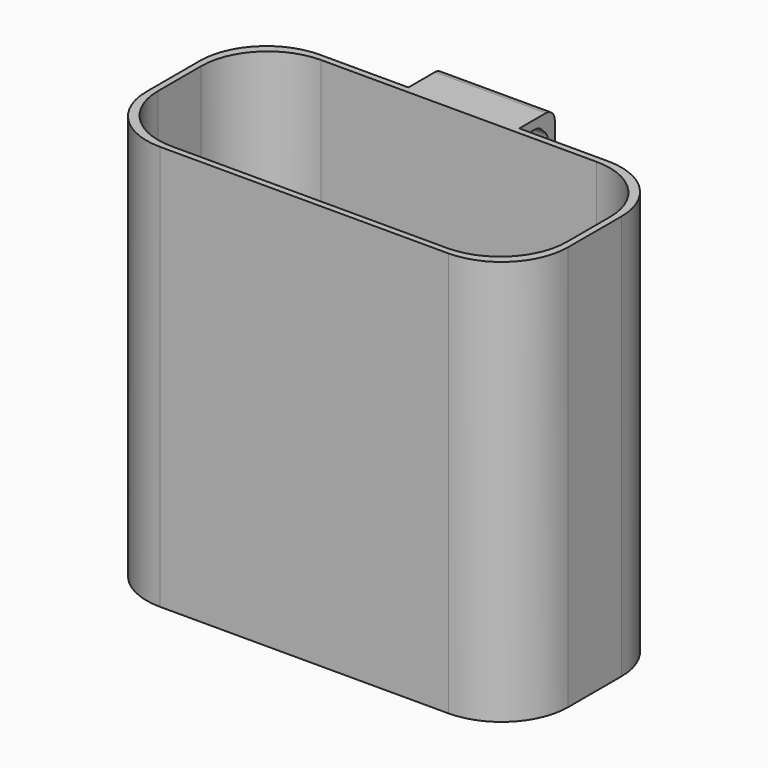
from build123d import *

# Parameters (mm, degrees)
F0_W          = 95
F0_H          = 45
F1_DEPTH      = 1.28
F2_W          = 95
F2_H          = 45
F2_W_2        = 92.12
F2_H_2        = 42.12
F3_DEPTH      = 90
F4_W          = 25
F4_H          = 35
F5_DEPTH      = 10
F6_W          = 8
F6_H          = 31
F7_DEPTH      = 60.001
F9_DEPTH      = 25
F11_DEPTH     = 10
F12_SIZE      = 2.5
F13_T1_DEPTH  = 25
F13_T3_DEPTH  = 37.5
F13_T5_DEPTH  = 28.3493649054
F13_T10_DEPTH = 35.1683904211
F13_T15_DEPTH = 35.1683904211
F14_R         = 15
F15_R         = 15
F16_R         = 15


# Not quite as in the source:
# - a fillet or chamfer that OpenCascade refuses, or shapes differently, is made with other operations: its cross-section is extruded or revolved along the edge and cut away or added


with BuildPart() as f1:
    # F0 (on Top) → F1 (new body)
    with BuildSketch(Plane.XY):
        with Locations((47.5, 22.5)):
            Rectangle(F0_W, F0_H)
    extrude(amount=F1_DEPTH)

    # F2 (on face) → F3 (join)
    with BuildSketch(Plane.XY.offset(1.28)):
        with Locations((47.5, 22.5)):
            Rectangle(F2_W, F2_H)
        with Locations((47.5, 22.5)):
            Rectangle(F2_W_2, F2_H_2, mode=Mode.SUBTRACT)
    extrude(amount=F3_DEPTH)

    # F4 (on face) → F5 (join)
    with BuildSketch(Plane(origin=(0, 45, 0), x_dir=(-1, 0, 0), z_dir=(0, 1, 0))):
        with Locations((-47.5, 73.78)):
            Rectangle(F4_W, F4_H)
    extrude(amount=F5_DEPTH)

    # F6 (on face) → F7 (cut, through all)
    with BuildSketch(Plane.YZ.offset(60)):
        with Locations((49, 73.78)):
            Rectangle(F6_W, F6_H)
    extrude(amount=-F7_DEPTH, mode=Mode.SUBTRACT)

    # F8 (on face) → F9 (join, through all)
    with BuildSketch(Plane.YZ.offset(60)):
        Polygon((55, 56.28), (45, 56.28), (45, 38.9594919243), align=None)
    extrude(amount=-F9_DEPTH)

    # F10 (on face) → F11 (cut, through all)
    with BuildSketch(Plane(origin=(0, 55, 0), x_dir=(-1, 0, 0), z_dir=(0, 1, 0))):
        Polygon((-53.6958506181, 38.9594919243), (-60, 56.28), (-60, 38.9594919243), align=None)
        Polygon((-41.304149382, 38.9594919243), (-35, 38.9594919243), (-35, 56.28), align=None)
    extrude(amount=-F11_DEPTH, mode=Mode.SUBTRACT)

    # F12
    f12_edges = [f1.edges().sort_by_distance(p)[0] for p in [
        (47.5, 45, 89.28),
        (47.5, 53, 89.28),
    ]]
    chamfer(f12_edges, length=F12_SIZE)

    # F13: fillet of radius 2.5 on 10 edges, made by hand

    # F13_s2 → F13_t1 (join)
    with BuildSketch(Plane.YZ.offset(35)):
        with BuildLine():
            ThreePointArc((45, 85.7444660941), (45.1903011687, 86.701174675), (45.732233047, 87.512233047))
            Line((45.732233047, 87.512233047), (45, 86.78))
            Line((45, 86.78), (45, 85.7444660941))
        make_face()
        with BuildLine():
            ThreePointArc((52.267766953, 87.512233047), (52.8096988313, 86.701174675), (53, 85.7444660941))
            Line((53, 85.7444660941), (53, 86.78))
            Line((53, 86.78), (52.267766953, 87.512233047))
        make_face()
        with BuildLine():
            ThreePointArc((50.5, 58.28), (52.267766953, 59.012233047), (53, 60.78))
            Line((53, 60.78), (53, 58.28))
            Line((53, 58.28), (50.5, 58.28))
        make_face()
        with BuildLine():
            ThreePointArc((45, 60.78), (45.732233047, 59.012233047), (47.5, 58.28))
            Line((47.5, 58.28), (45, 58.28))
            Line((45, 58.28), (45, 60.78))
        make_face()
        with BuildLine():
            ThreePointArc((46.767766953, 88.547766953), (47.578825325, 89.0896988313), (48.5355339059, 89.28))
            Line((48.5355339059, 89.28), (47.5, 89.28))
            Line((47.5, 89.28), (46.767766953, 88.547766953))
        make_face()
        with BuildLine():
            ThreePointArc((49.4644660941, 89.28), (50.421174675, 89.0896988313), (51.232233047, 88.547766953))
            Line((51.232233047, 88.547766953), (50.5, 89.28))
            Line((50.5, 89.28), (49.4644660941, 89.28))
        make_face()
    extrude(amount=F13_T1_DEPTH)

    # F13_s4 → F13_t3 (cut)
    with BuildSketch(Plane.YZ.offset(28.75)):
        with BuildLine():
            ThreePointArc((55, 88.78), (54.267766953, 90.547766953), (52.5, 91.28))
            Line((52.5, 91.28), (55, 91.28))
            Line((55, 91.28), (55, 88.78))
        make_face()
    extrude(amount=F13_T3_DEPTH, mode=Mode.SUBTRACT)

    # F13_s6 → F13_t5 (cut)
    with BuildSketch(Plane.YZ.offset(33.3253175473)):
        with BuildLine():
            ThreePointArc((54.6650635095, 55.6998729811), (54.9148145657, 56.3028253683), (55, 56.9498729811))
            Line((55, 56.9498729811), (55, 56.28))
            Line((55, 56.28), (54.6650635095, 55.6998729811))
        make_face()
    extrude(amount=F13_T5_DEPTH, mode=Mode.SUBTRACT)


with BuildPart() as f13_tool8:
    # F13_s9 → F13_t10 (new body)
    with BuildSketch(Plane(origin=(19.397060828, 30.7687201759, 53.2929866286), x_dir=(-0.8459331757, 0.5332889107, 0), z_dir=(0.3006265785, 0.4768709627, 0.8259647361))):
        with BuildLine():
            ThreePointArc((-19.5594103687, -32.1600455029), (-21.2581254439, -32.3827100323), (-22.7013076364, -31.4594345813))
            Line((-22.7013076364, -31.4594345813), (-21.425100455, -33.1315112786))
            Line((-21.425100455, -33.1315112786), (-19.5594103687, -32.1600455029))
        make_face()
    extrude(amount=F13_T10_DEPTH)

    split(bisect_by=Plane.XZ.offset(-45), keep=Keep.BOTTOM)


with BuildPart() as f1_1:
    add(f1.part)

    # F13_t7: cut F13_tool8
    add(f13_tool8.part, mode=Mode.SUBTRACT)


with BuildPart() as f13_tool13:
    # F13_s14 → F13_t15 (new body)
    with BuildSketch(Plane(origin=(-21.3838614404, 33.9202962128, 58.7516764483), x_dir=(0.8459331757, 0.5332889107, 0), z_dir=(0.3006265785, -0.4768709627, -0.8259647361))):
        with BuildLine():
            ThreePointArc((57.6623440552, 10.3859596823), (59.1055262478, 9.4626842314), (60.8042413229, 9.6853487608))
            Line((60.8042413229, 9.6853487608), (58.9385512366, 8.713882985))
            Line((58.9385512366, 8.713882985), (57.6623440552, 10.3859596823))
        make_face()
    extrude(amount=F13_T15_DEPTH)

    split(bisect_by=Plane.XZ.offset(-45), keep=Keep.BOTTOM)


with BuildPart() as f1_2:
    add(f1_1.part)

    # F13_t12: cut F13_tool13
    add(f13_tool13.part, mode=Mode.SUBTRACT)

    # F14
    f14_edges = [f1_2.edges().sort_by_distance(p)[0] for p in [
        (1.44, 43.56, 46.28),
        (1.44, 1.44, 46.28),
        (93.56, 43.56, 46.28),
        (93.56, 1.44, 46.28),
    ]]
    fillet(f14_edges, radius=F14_R)

    # F15
    f15_edges = [f1_2.edges().sort_by_distance(p)[0] for p in [
        (95, 0, 45.64),
        (95, 45, 45.64),
        (0, 45, 45.64),
        (0, 0, 45.64),
    ]]
    fillet(f15_edges, radius=F15_R)

    # F16
    f16_edges = [f1_2.edges().sort_by_distance(p)[0] for p in [
        (47.5, 43.56, 1.28),
        (5.833398, 39.166602, 1.28),
        (89.166602, 39.166602, 1.28),
        (1.44, 22.5, 1.28),
        (93.56, 22.5, 1.28),
        (5.833398, 5.833398, 1.28),
        (89.166602, 5.833398, 1.28),
        (47.5, 1.44, 1.28),
    ]]
    fillet(f16_edges, radius=F16_R)


solid = f1_2.part
